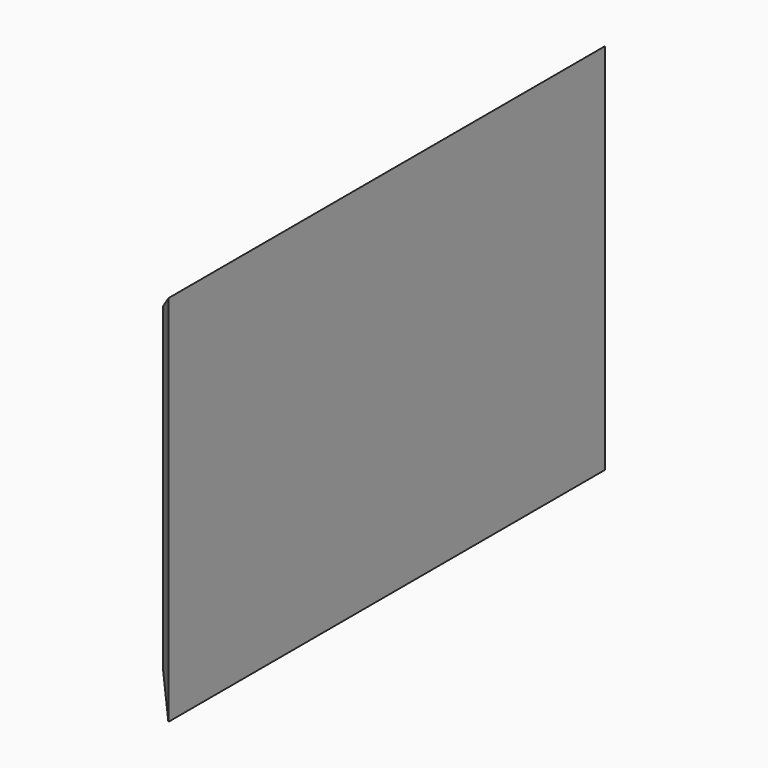
from build123d import *

# Parameters (mm, degrees)
F0_W     = 381
F0_H     = 260.35
F1_DEPTH = 19.05
F2_SIZE  = 19.04999


# Not quite as in the source:
# - a fillet or chamfer is up to 0.001 mm smaller than in the source, because OpenCascade refuses the exact size


with BuildPart() as f1:
    # F0 (on Right) → F1 (new body)
    with BuildSketch(Plane.YZ):
        Rectangle(F0_W, F0_H)
    extrude(amount=F1_DEPTH)

    # F2 (size 19.05 in the source; OpenCascade refuses exactly that, so slightly less here)
    f2_edges = [f1.edges().sort_by_distance(p)[0] for p in [
        (0, 0, -130.175),
        (0, 0, 130.175),
        (0, -190.5, 0),
    ]]
    chamfer(f2_edges, length=F2_SIZE)


solid = f1.part
